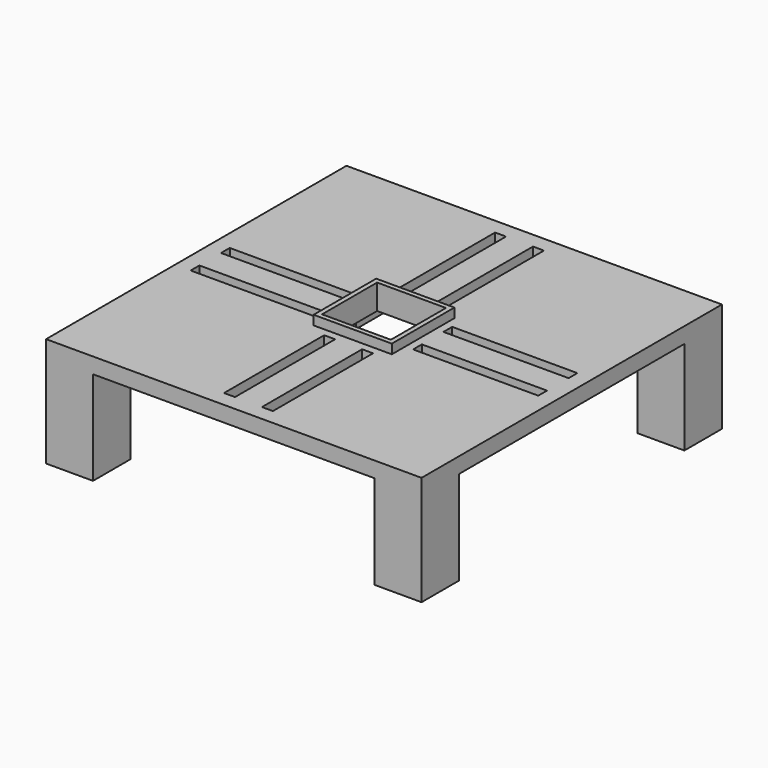
from build123d import *

# Parameters (mm, degrees)
F0_W             = 120
F0_H             = 120
F1_DEPTH         = 5
F2_W             = 15
F2_H             = 15
F3_DEPTH         = 30
F4_W             = 10
F4_H             = 10
F5_DEPTH         = 10
F6_W             = 25
F6_H             = 25
F7_DEPTH         = 3
F8_W             = 22
F8_H             = 22
F9_DEPTH         = 8
F10_W            = 3.5
F10_H            = 40
F11_DEPTH        = 5
F11_COPIES_COUNT = 4
F13_W            = 6.5
F13_H            = 42.5
F14_DEPTH        = 2
F14_COPIES_COUNT = 4


# Not quite as in the source:
# - a pattern or mirror of a feature is missing from the dataset's text; its kind, count and spacing are read off the source's solid


with BuildPart() as f1:
    # F0 (on Top) → F1 (new body)
    with BuildSketch(Plane.XY):
        Rectangle(F0_W, F0_H)
    extrude(amount=-F1_DEPTH)

    # F2 (on face) → F3 (join)
    with BuildSketch(Plane(origin=(0, 0, -5), x_dir=(1, 0, 0), z_dir=(0, 0, -1))):
        with Locations((-52.5, 52.5)):
            Rectangle(F2_W, F2_H)
        with Locations((-52.5, -52.5)):
            Rectangle(F2_W, F2_H)
        with Locations((52.5, -52.5)):
            Rectangle(F2_W, F2_H)
        with Locations((52.5, 52.5)):
            Rectangle(F2_W, F2_H)
    extrude(amount=F3_DEPTH)

    # F4 (on face) → F5 (cut)
    with BuildSketch(Plane(origin=(0, 0, -35), x_dir=(1, 0, 0), z_dir=(0, 0, -1))):
        with Locations((-52.5, 52.5)):
            Rectangle(F4_W, F4_H)
        with Locations((-52.5, -52.5)):
            Rectangle(F4_W, F4_H)
        with Locations((52.5, -52.5)):
            Rectangle(F4_W, F4_H)
        with Locations((52.5, 52.5)):
            Rectangle(F4_W, F4_H)
    extrude(amount=-F5_DEPTH, mode=Mode.SUBTRACT)

    # F6 (on face) → F7 (join)
    with BuildSketch(Plane.XY):
        Rectangle(F6_W, F6_H)
    extrude(amount=F7_DEPTH)

    # F8 (on face) → F9 (cut, through all)
    with BuildSketch(Plane.XY.offset(3)):
        Rectangle(F8_W, F8_H)
    extrude(amount=-F9_DEPTH, mode=Mode.SUBTRACT)

    # F10 (on face) → F11 (cut, through all)
    with BuildSketch(Plane(origin=(0, 0, -5), x_dir=(1, 0, 0), z_dir=(0, 0, -1))):
        with Locations((-6.75, -35)):
            Rectangle(F10_W, F10_H)
        with Locations((5.3777624313, -35)):
            Rectangle(F10_W, F10_H)
    f11 = extrude(amount=-F11_DEPTH, mode=Mode.SUBTRACT)

    # F11_copies: F11 ×4 about axis
    f11_copies_axis = Axis((0, 0, 0), (0, 0, 1))
    for i in range(1, F11_COPIES_COUNT):
        add(f11.rotate(f11_copies_axis, i * 360 / F11_COPIES_COUNT), mode=Mode.SUBTRACT)

    # F13 (on face) → F14 (cut)
    with BuildSketch(Plane(origin=(0, 0, -5), x_dir=(1, 0, 0), z_dir=(0, 0, -1))):
        with Locations((5.3777624313, -35.25)):
            Rectangle(F13_W, F13_H)
        with Locations((-6.75, -35.25)):
            Rectangle(F13_W, F13_H)
    f14 = extrude(amount=-F14_DEPTH, mode=Mode.SUBTRACT)

    # F14_copies: F14 ×4 about axis
    f14_copies_axis = Axis((0, 0, 0), (0, 0, 1))
    for i in range(1, F14_COPIES_COUNT):
        add(f14.rotate(f14_copies_axis, i * 360 / F14_COPIES_COUNT), mode=Mode.SUBTRACT)


solid = f1.part
